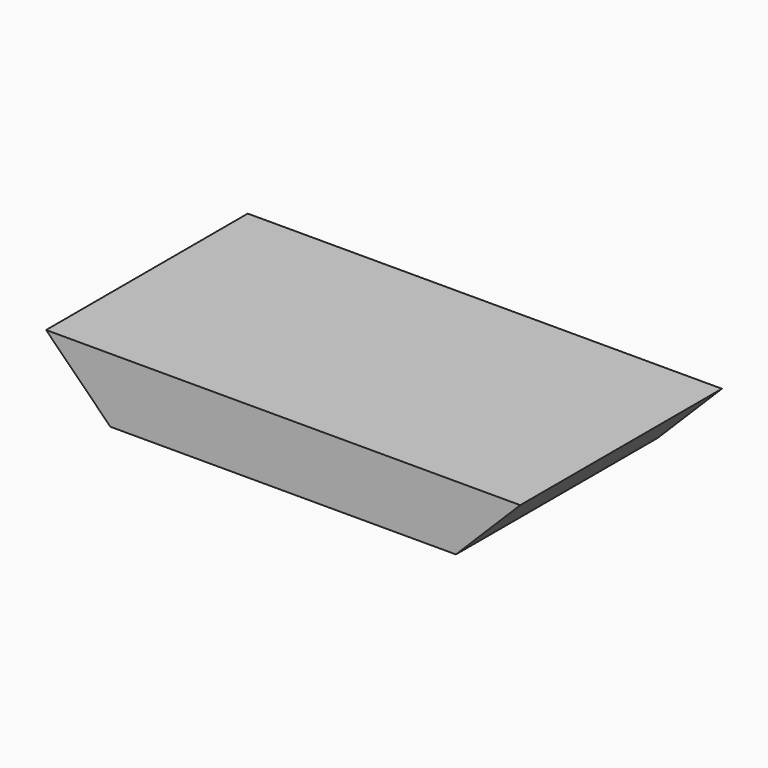
from build123d import *

# Parameters (mm, degrees)
F0_W     = 187.2611194849
F0_H     = 99.5552539825
F1_DEPTH = 25.4
F2_SIZE  = 25.39999


# Not quite as in the source:
# - a fillet or chamfer is up to 0.001 mm smaller than in the source, because OpenCascade refuses the exact size


with BuildPart() as f1:
    # F0 (on Top) → F1 (new body)
    with BuildSketch(Plane.XY):
        Rectangle(F0_W, F0_H)
    extrude(amount=F1_DEPTH)

    # F2 (size 25.4 in the source; OpenCascade refuses exactly that, so slightly less here)
    f2_edges = [f1.edges().sort_by_distance(p)[0] for p in [
        (-93.63056, 0, 0),
        (93.63056, 0, 0),
    ]]
    chamfer(f2_edges, length=F2_SIZE)


solid = f1.part
